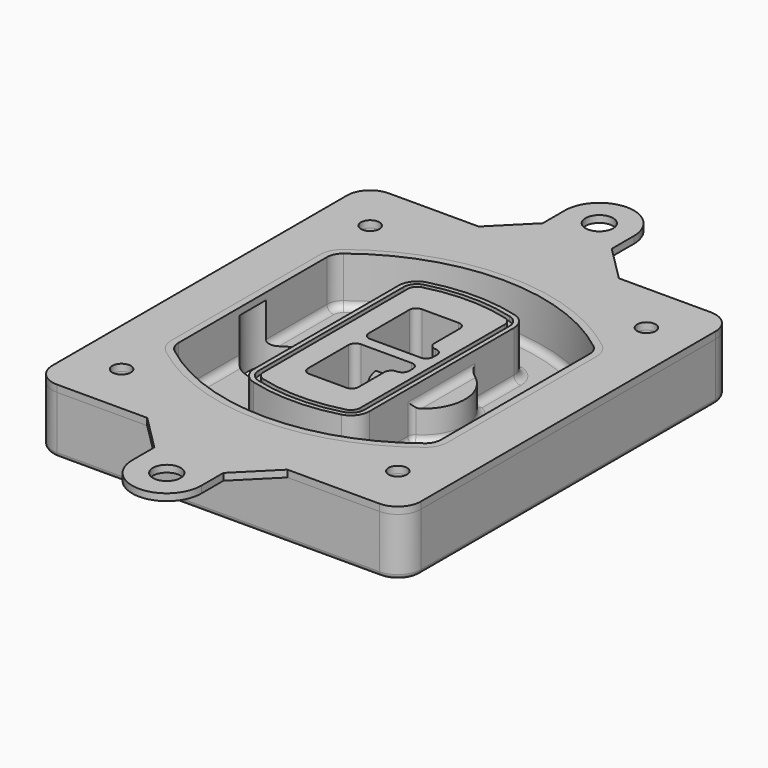
from build123d import *

# Parameters (mm, degrees)
F0_R      = 4
F1_DEPTH  = 25
F2_DEPTH  = 3
F3_DEPTH  = 18
F5_DEPTH  = 21
F6_DEPTH  = 2
F8_DEPTH  = 20
F9_DEPTH  = 16
F10_DEPTH = 25
F7_R      = 6
F7_R_2    = 4
F11_DEPTH = 6
F13_DEPTH = 9
F14_R     = 3
F15_R     = 2
F16_R     = 4
F16_R_2   = 6
F17_DEPTH = 3


# Not quite as in the source:
# - a feature names something its author has since deleted; it is built from what else it names


with BuildPart() as f1:
    # F0 (on Top) → F1 (new body)
    with BuildSketch(Plane.XY):
        with BuildLine():
            ThreePointArc((-80, -80), (-77.0710678119, -87.0710678119), (-70, -90))
            Line((-70, -90), (70, -90))
            ThreePointArc((70, -90), (77.0710678119, -87.0710678119), (80, -80))
            Line((80, -80), (80, 80))
            ThreePointArc((80, 80), (77.0710678119, 87.0710678119), (70, 90))
            Line((70, 90), (-70, 90))
            ThreePointArc((-70, 90), (-77.0710678119, 87.0710678119), (-80, 80))
            Line((-80, 80), (-80, -80))
        make_face()
        with Locations((-60, -67.5)):
            Circle(F0_R, mode=Mode.SUBTRACT)
        with Locations((60, -67.5)):
            Circle(F0_R, mode=Mode.SUBTRACT)
        with Locations((-60, 67.5)):
            Circle(F0_R, mode=Mode.SUBTRACT)
        with BuildLine():
            ThreePointArc((-64, 40.2934422872), (-62.5820384798, 46.4328484224), (-58.6153846154, 51.3286200352))
            ThreePointArc((-58.6153846154, 51.3286200352), (0, 71.5), (58.6153846154, 51.3286200352))
            ThreePointArc((58.6153846154, 51.3286200352), (62.5820384798, 46.4328484224), (64, 40.2934422872))
            Line((64, 40.2934422872), (64, -40.2934422872))
            ThreePointArc((64, -40.2934422872), (62.5820384798, -46.4328484224), (58.6153846154, -51.3286200352))
            ThreePointArc((58.6153846154, -51.3286200352), (0, -71.5), (-58.6153846154, -51.3286200352))
            ThreePointArc((-58.6153846154, -51.3286200352), (-62.5820384798, -46.4328484224), (-64, -40.2934422872))
            Line((-64, -40.2934422872), (-64, 40.2934422872))
        make_face(mode=Mode.SUBTRACT)
        with Locations((60, 67.5)):
            Circle(F0_R, mode=Mode.SUBTRACT)
        with BuildLine():
            ThreePointArc((58.6153846154, 51.3286200352), (0, 71.5), (-58.6153846154, 51.3286200352))
            ThreePointArc((-58.6153846154, 51.3286200352), (-62.5820384798, 46.4328484224), (-64, 40.2934422872))
            Line((-64, 40.2934422872), (-64, -40.2934422872))
            ThreePointArc((-64, -40.2934422872), (-62.5820384798, -46.4328484224), (-58.6153846154, -51.3286200352))
            ThreePointArc((-58.6153846154, -51.3286200352), (0, -71.5), (58.6153846154, -51.3286200352))
            ThreePointArc((58.6153846154, -51.3286200352), (62.5820384798, -46.4328484224), (64, -40.2934422872))
            Line((64, -40.2934422872), (64, 40.2934422872))
            ThreePointArc((64, 40.2934422872), (62.5820384798, 46.4328484224), (58.6153846154, 51.3286200352))
        make_face()
        with BuildLine():
            Line((-60, -40.2934422872), (-60, 40.2934422872))
            ThreePointArc((-60, 40.2934422872), (-58.9871703427, 44.6787323838), (-56.1538461538, 48.1757121072))
            ThreePointArc((-56.1538461538, 48.1757121072), (0, 67.5), (56.1538461538, 48.1757121072))
            ThreePointArc((56.1538461538, 48.1757121072), (58.9871703427, 44.6787323838), (60, 40.2934422872))
            Line((60, 40.2934422872), (60, -40.2934422872))
            ThreePointArc((60, -40.2934422872), (58.9871703427, -44.6787323838), (56.1538461538, -48.1757121072))
            ThreePointArc((56.1538461538, -48.1757121072), (0, -67.5), (-56.1538461538, -48.1757121072))
            ThreePointArc((-56.1538461538, -48.1757121072), (-58.9871703427, -44.6787323838), (-60, -40.2934422872))
        make_face(mode=Mode.SUBTRACT)
        with BuildLine():
            ThreePointArc((-56.1538461538, 48.1757121072), (-58.9871703427, 44.6787323838), (-60, 40.2934422872))
            Line((-60, 40.2934422872), (-60, -40.2934422872))
            ThreePointArc((-60, -40.2934422872), (-58.9871703427, -44.6787323838), (-56.1538461538, -48.1757121072))
            ThreePointArc((-56.1538461538, -48.1757121072), (0, -67.5), (56.1538461538, -48.1757121072))
            ThreePointArc((56.1538461538, -48.1757121072), (58.9871703427, -44.6787323838), (60, -40.2934422872))
            Line((60, -40.2934422872), (60, 40.2934422872))
            ThreePointArc((60, 40.2934422872), (58.9871703427, 44.6787323838), (56.1538461538, 48.1757121072))
            ThreePointArc((56.1538461538, 48.1757121072), (0, 67.5), (-56.1538461538, 48.1757121072))
        make_face()
        with BuildLine():
            ThreePointArc((54.3076923077, 45.8110311612), (56.2910192399, 43.3631453548), (57, 40.2934422872))
            Line((57, 40.2934422872), (57, -40.2934422872))
            ThreePointArc((57, -40.2934422872), (56.2910192399, -43.3631453548), (54.3076923077, -45.8110311612))
            ThreePointArc((54.3076923077, -45.8110311612), (0, -64.5), (-54.3076923077, -45.8110311612))
            ThreePointArc((-54.3076923077, -45.8110311612), (-56.2910192399, -43.3631453548), (-57, -40.2934422872))
            Line((-57, -40.2934422872), (-57, 40.2934422872))
            ThreePointArc((-57, 40.2934422872), (-56.2910192399, 43.3631453548), (-54.3076923077, 45.8110311612))
            ThreePointArc((-54.3076923077, 45.8110311612), (0, 64.5), (54.3076923077, 45.8110311612))
        make_face(mode=Mode.SUBTRACT)
        with BuildLine():
            Line((57, -40.2934422872), (57, 40.2934422872))
            ThreePointArc((57, 40.2934422872), (56.2910192399, 43.3631453548), (54.3076923077, 45.8110311612))
            ThreePointArc((54.3076923077, 45.8110311612), (0, 64.5), (-54.3076923077, 45.8110311612))
            ThreePointArc((-54.3076923077, 45.8110311612), (-56.2910192399, 43.3631453548), (-57, 40.2934422872))
            Line((-57, 40.2934422872), (-57, -40.2934422872))
            ThreePointArc((-57, -40.2934422872), (-56.2910192399, -43.3631453548), (-54.3076923077, -45.8110311612))
            ThreePointArc((-54.3076923077, -45.8110311612), (0, -64.5), (54.3076923077, -45.8110311612))
            ThreePointArc((54.3076923077, -45.8110311612), (56.2910192399, -43.3631453548), (57, -40.2934422872))
        make_face()
    extrude(amount=-F1_DEPTH)

    # F0 (on Top) → F2 (join)
    with BuildSketch(Plane.XY):
        with BuildLine():
            ThreePointArc((-56.1538461538, 48.1757121072), (-58.9871703427, 44.6787323838), (-60, 40.2934422872))
            Line((-60, 40.2934422872), (-60, -40.2934422872))
            ThreePointArc((-60, -40.2934422872), (-58.9871703427, -44.6787323838), (-56.1538461538, -48.1757121072))
            ThreePointArc((-56.1538461538, -48.1757121072), (0, -67.5), (56.1538461538, -48.1757121072))
            ThreePointArc((56.1538461538, -48.1757121072), (58.9871703427, -44.6787323838), (60, -40.2934422872))
            Line((60, -40.2934422872), (60, 40.2934422872))
            ThreePointArc((60, 40.2934422872), (58.9871703427, 44.6787323838), (56.1538461538, 48.1757121072))
            ThreePointArc((56.1538461538, 48.1757121072), (0, 67.5), (-56.1538461538, 48.1757121072))
        make_face()
        with BuildLine():
            ThreePointArc((54.3076923077, 45.8110311612), (56.2910192399, 43.3631453548), (57, 40.2934422872))
            Line((57, 40.2934422872), (57, -40.2934422872))
            ThreePointArc((57, -40.2934422872), (56.2910192399, -43.3631453548), (54.3076923077, -45.8110311612))
            ThreePointArc((54.3076923077, -45.8110311612), (0, -64.5), (-54.3076923077, -45.8110311612))
            ThreePointArc((-54.3076923077, -45.8110311612), (-56.2910192399, -43.3631453548), (-57, -40.2934422872))
            Line((-57, -40.2934422872), (-57, 40.2934422872))
            ThreePointArc((-57, 40.2934422872), (-56.2910192399, 43.3631453548), (-54.3076923077, 45.8110311612))
            ThreePointArc((-54.3076923077, 45.8110311612), (0, 64.5), (54.3076923077, 45.8110311612))
        make_face(mode=Mode.SUBTRACT)
    extrude(amount=F2_DEPTH)

    # F0 (on Top) → F3 (cut)
    with BuildSketch(Plane.XY):
        with BuildLine():
            Line((57, -40.2934422872), (57, 40.2934422872))
            ThreePointArc((57, 40.2934422872), (56.2910192399, 43.3631453548), (54.3076923077, 45.8110311612))
            ThreePointArc((54.3076923077, 45.8110311612), (0, 64.5), (-54.3076923077, 45.8110311612))
            ThreePointArc((-54.3076923077, 45.8110311612), (-56.2910192399, 43.3631453548), (-57, 40.2934422872))
            Line((-57, 40.2934422872), (-57, -40.2934422872))
            ThreePointArc((-57, -40.2934422872), (-56.2910192399, -43.3631453548), (-54.3076923077, -45.8110311612))
            ThreePointArc((-54.3076923077, -45.8110311612), (0, -64.5), (54.3076923077, -45.8110311612))
            ThreePointArc((54.3076923077, -45.8110311612), (56.2910192399, -43.3631453548), (57, -40.2934422872))
        make_face()
    extrude(amount=-F3_DEPTH, mode=Mode.SUBTRACT)

    # F4 (on face) → F5 (join, through all)
    with BuildSketch(Plane.XY.offset(3)):
        with BuildLine():
            ThreePointArc((-25, -39.2465276821), (-23.3511545998, -44.1109737193), (-19.0842911877, -46.9702398883))
            ThreePointArc((-19.0842911877, -46.9702398883), (0, -49.5), (19.0842911877, -46.9702398883))
            ThreePointArc((19.0842911877, -46.9702398883), (23.3511545998, -44.1109737193), (25, -39.2465276821))
            Line((25, -39.2465276821), (25, 39.2465276821))
            ThreePointArc((25, 39.2465276821), (23.3511545998, 44.1109737193), (19.0842911877, 46.9702398883))
            ThreePointArc((19.0842911877, 46.9702398883), (0, 49.5), (-19.0842911877, 46.9702398883))
            ThreePointArc((-19.0842911877, 46.9702398883), (-23.3511545998, 44.1109737193), (-25, 39.2465276821))
            Line((-25, 39.2465276821), (-25, -39.2465276821))
        make_face()
        with BuildLine():
            ThreePointArc((18.5632183908, 45.0393118368), (21.7633659499, 42.89486221), (23, 39.2465276821))
            Line((23, 39.2465276821), (23, -39.2465276821))
            ThreePointArc((23, -39.2465276821), (21.7633659499, -42.89486221), (18.5632183908, -45.0393118368))
            ThreePointArc((18.5632183908, -45.0393118368), (0, -47.5), (-18.5632183908, -45.0393118368))
            ThreePointArc((-18.5632183908, -45.0393118368), (-21.7633659499, -42.89486221), (-23, -39.2465276821))
            Line((-23, -39.2465276821), (-23, 39.2465276821))
            ThreePointArc((-23, 39.2465276821), (-21.7633659499, 42.89486221), (-18.5632183908, 45.0393118368))
            ThreePointArc((-18.5632183908, 45.0393118368), (0, 47.5), (18.5632183908, 45.0393118368))
        make_face(mode=Mode.SUBTRACT)
        with BuildLine():
            Line((23, -39.2465276821), (23, 39.2465276821))
            ThreePointArc((23, 39.2465276821), (21.7633659499, 42.89486221), (18.5632183908, 45.0393118368))
            ThreePointArc((18.5632183908, 45.0393118368), (0, 47.5), (-18.5632183908, 45.0393118368))
            ThreePointArc((-18.5632183908, 45.0393118368), (-21.7633659499, 42.89486221), (-23, 39.2465276821))
            Line((-23, 39.2465276821), (-23, -39.2465276821))
            ThreePointArc((-23, -39.2465276821), (-21.7633659499, -42.89486221), (-18.5632183908, -45.0393118368))
            ThreePointArc((-18.5632183908, -45.0393118368), (0, -47.5), (18.5632183908, -45.0393118368))
            ThreePointArc((18.5632183908, -45.0393118368), (21.7633659499, -42.89486221), (23, -39.2465276821))
        make_face()
        with BuildLine():
            ThreePointArc((18.0421455939, 43.1083837852), (20.1755772999, 41.6787507007), (21, 39.2465276821))
            Line((21, 39.2465276821), (21, -39.2465276821))
            ThreePointArc((21, -39.2465276821), (20.1755772999, -41.6787507007), (18.0421455939, -43.1083837852))
            ThreePointArc((18.0421455939, -43.1083837852), (0, -45.5), (-18.0421455939, -43.1083837852))
            ThreePointArc((-18.0421455939, -43.1083837852), (-20.1755772999, -41.6787507007), (-21, -39.2465276821))
            Line((-21, -39.2465276821), (-21, 39.2465276821))
            ThreePointArc((-21, 39.2465276821), (-20.1755772999, 41.6787507007), (-18.0421455939, 43.1083837852))
            ThreePointArc((-18.0421455939, 43.1083837852), (0, 45.5), (18.0421455939, 43.1083837852))
        make_face(mode=Mode.SUBTRACT)
        with BuildLine():
            Line((21, -39.2465276821), (21, 39.2465276821))
            ThreePointArc((21, 39.2465276821), (20.1755772999, 41.6787507007), (18.0421455939, 43.1083837852))
            ThreePointArc((18.0421455939, 43.1083837852), (0, 45.5), (-18.0421455939, 43.1083837852))
            ThreePointArc((-18.0421455939, 43.1083837852), (-20.1755772999, 41.6787507007), (-21, 39.2465276821))
            Line((-21, 39.2465276821), (-21, -39.2465276821))
            ThreePointArc((-21, -39.2465276821), (-20.1755772999, -41.6787507007), (-18.0421455939, -43.1083837852))
            ThreePointArc((-18.0421455939, -43.1083837852), (0, -45.5), (18.0421455939, -43.1083837852))
            ThreePointArc((18.0421455939, -43.1083837852), (20.1755772999, -41.6787507007), (21, -39.2465276821))
        make_face()
        with BuildLine():
            Line((-8, -2.5), (14, -2.5))
            ThreePointArc((14, -2.5), (16.1213203436, -3.3786796564), (17, -5.5))
            Line((17, -5.5), (17, -7.5))
            ThreePointArc((17, -7.5), (16.1213203436, -9.6213203436), (14, -10.5))
            ThreePointArc((14, -10.5), (11.8786796564, -11.3786796564), (11, -13.5))
            Line((11, -13.5), (11, -27.5))
            ThreePointArc((11, -27.5), (10.1213203436, -29.6213203436), (8, -30.5))
            Line((8, -30.5), (-8, -30.5))
            ThreePointArc((-8, -30.5), (-10.1213203436, -29.6213203436), (-11, -27.5))
            Line((-11, -27.5), (-11, -5.5))
            ThreePointArc((-11, -5.5), (-10.1213203436, -3.3786796564), (-8, -2.5))
        make_face(mode=Mode.SUBTRACT)
        with BuildLine():
            ThreePointArc((-8, 2.5), (-10.1213203436, 3.3786796564), (-11, 5.5))
            Line((-11, 5.5), (-11, 27.5))
            ThreePointArc((-11, 27.5), (-10.1213203436, 29.6213203436), (-8, 30.5))
            Line((-8, 30.5), (8, 30.5))
            ThreePointArc((8, 30.5), (10.1213203436, 29.6213203436), (11, 27.5))
            Line((11, 27.5), (11, 13.5))
            ThreePointArc((11, 13.5), (11.8786796564, 11.3786796564), (14, 10.5))
            ThreePointArc((14, 10.5), (16.1213203436, 9.6213203436), (17, 7.5))
            Line((17, 7.5), (17, 5.5))
            ThreePointArc((17, 5.5), (16.1213203436, 3.3786796564), (14, 2.5))
            Line((14, 2.5), (-8, 2.5))
        make_face(mode=Mode.SUBTRACT)
    extrude(amount=-F5_DEPTH)

    # F4 (on face) → F6 (cut)
    with BuildSketch(Plane.XY.offset(3)):
        with BuildLine():
            Line((23, -39.2465276821), (23, 39.2465276821))
            ThreePointArc((23, 39.2465276821), (21.7633659499, 42.89486221), (18.5632183908, 45.0393118368))
            ThreePointArc((18.5632183908, 45.0393118368), (0, 47.5), (-18.5632183908, 45.0393118368))
            ThreePointArc((-18.5632183908, 45.0393118368), (-21.7633659499, 42.89486221), (-23, 39.2465276821))
            Line((-23, 39.2465276821), (-23, -39.2465276821))
            ThreePointArc((-23, -39.2465276821), (-21.7633659499, -42.89486221), (-18.5632183908, -45.0393118368))
            ThreePointArc((-18.5632183908, -45.0393118368), (0, -47.5), (18.5632183908, -45.0393118368))
            ThreePointArc((18.5632183908, -45.0393118368), (21.7633659499, -42.89486221), (23, -39.2465276821))
        make_face()
        with BuildLine():
            ThreePointArc((18.0421455939, 43.1083837852), (20.1755772999, 41.6787507007), (21, 39.2465276821))
            Line((21, 39.2465276821), (21, -39.2465276821))
            ThreePointArc((21, -39.2465276821), (20.1755772999, -41.6787507007), (18.0421455939, -43.1083837852))
            ThreePointArc((18.0421455939, -43.1083837852), (0, -45.5), (-18.0421455939, -43.1083837852))
            ThreePointArc((-18.0421455939, -43.1083837852), (-20.1755772999, -41.6787507007), (-21, -39.2465276821))
            Line((-21, -39.2465276821), (-21, 39.2465276821))
            ThreePointArc((-21, 39.2465276821), (-20.1755772999, 41.6787507007), (-18.0421455939, 43.1083837852))
            ThreePointArc((-18.0421455939, 43.1083837852), (0, 45.5), (18.0421455939, 43.1083837852))
        make_face(mode=Mode.SUBTRACT)
    extrude(amount=-F6_DEPTH, mode=Mode.SUBTRACT)

    # F7 (on face) → F8 (join)
    with BuildSketch(Plane(origin=(0, 0, -25), x_dir=(1, 0, 0), z_dir=(0, 0, -1))):
        with BuildLine():
            ThreePointArc((3.28842436, 0), (16.7567035675, 13.4682792075), (30.224982775, 0))
            Line((30.224982775, 0), (35.224982775, 0))
            ThreePointArc((35.224982775, 0), (16.7567035675, 18.4682792075), (-1.71157564, 0))
            Line((-1.71157564, 0), (3.28842436, 0))
        make_face()
        with BuildLine():
            Line((3.28842436, 0), (30.224982775, 0))
            ThreePointArc((30.224982775, 0), (16.7567035675, 13.4682792075), (3.28842436, 0))
        make_face()
        with BuildLine():
            ThreePointArc((3.28842436, 0), (16.7567035675, -13.4682792075), (30.224982775, 0))
            Line((30.224982775, 0), (3.28842436, 0))
        make_face()
        with BuildLine():
            Line((35.224982775, 0), (30.224982775, 0))
            ThreePointArc((30.224982775, 0), (16.7567035675, -13.4682792075), (3.28842436, 0))
            Line((3.28842436, 0), (-1.71157564, 0))
            ThreePointArc((-1.71157564, 0), (16.7567035675, -18.4682792075), (35.224982775, 0))
        make_face()
    extrude(amount=-F8_DEPTH)

    # F7 (on face) → F9 (cut)
    with BuildSketch(Plane(origin=(0, 0, -25), x_dir=(1, 0, 0), z_dir=(0, 0, -1))):
        with BuildLine():
            Line((3.28842436, 0), (30.224982775, 0))
            ThreePointArc((30.224982775, 0), (16.7567035675, 13.4682792075), (3.28842436, 0))
        make_face()
        with BuildLine():
            ThreePointArc((3.28842436, 0), (16.7567035675, -13.4682792075), (30.224982775, 0))
            Line((30.224982775, 0), (3.28842436, 0))
        make_face()
    extrude(amount=-F9_DEPTH, mode=Mode.SUBTRACT)

    # F7 (on face) → F10 (cut)
    with BuildSketch(Plane(origin=(0, 0, -25), x_dir=(1, 0, 0), z_dir=(0, 0, -1))):
        with BuildLine():
            Line((-59.0318229325, 0), (-32.0952645175, 0))
            ThreePointArc((-32.0952645175, 0), (-45.563543725, 13.4682792075), (-59.0318229325, 0))
        make_face()
        with BuildLine():
            ThreePointArc((-59.0318229325, 0), (-45.563543725, -13.4682792075), (-32.0952645175, 0))
            Line((-32.0952645175, 0), (-59.0318229325, 0))
        make_face()
    extrude(amount=-F10_DEPTH, mode=Mode.SUBTRACT)

    # F7 (on face) → F11 (cut)
    with BuildSketch(Plane(origin=(0, 0, -25), x_dir=(1, 0, 0), z_dir=(0, 0, -1))):
        with Locations((60, -67.5)):
            Circle(F7_R)
        with Locations((60, -67.5)):
            Circle(F7_R_2, mode=Mode.SUBTRACT)
        with Locations((-60, -67.5)):
            Circle(F7_R)
        with Locations((-60, -67.5)):
            Circle(F7_R_2, mode=Mode.SUBTRACT)
        with Locations((-60, 67.5)):
            Circle(F7_R)
        with Locations((-60, 67.5)):
            Circle(F7_R_2, mode=Mode.SUBTRACT)
        with Locations((60, 67.5)):
            Circle(F7_R)
        with Locations((60, 67.5)):
            Circle(F7_R_2, mode=Mode.SUBTRACT)
    extrude(amount=-F11_DEPTH, mode=Mode.SUBTRACT)

    # F12 (on face) → F13 (cut, through all)
    with BuildSketch(Plane(origin=(0, 0, -9), x_dir=(1, 0, 0), z_dir=(0, 0, -1))):
        with BuildLine():
            Line((11, 13.5), (11, 17.5481537753))
            ThreePointArc((11, 17.5481537753), (2.5696536419, 11.8239143813), (-1.5415842455, 2.5))
            Line((-1.5415842455, 2.5), (3.5224848595, 2.5))
            ThreePointArc((3.5224848595, 2.5), (6.1857188154, 8.3455872281), (11.2536447004, 12.2927168648))
            ThreePointArc((11.2536447004, 12.2927168648), (11.0640958889, 12.8831798879), (11, 13.5))
        make_face()
        with BuildLine():
            ThreePointArc((11.2536447004, -12.2927168648), (6.1857188154, -8.3455872281), (3.5224848595, -2.5))
            Line((3.5224848595, -2.5), (-1.5415842455, -2.5))
            ThreePointArc((-1.5415842455, -2.5), (2.5696536419, -11.8239143813), (11, -17.5481537753))
            Line((11, -17.5481537753), (11, -13.5))
            ThreePointArc((11, -13.5), (11.0640958889, -12.8831798879), (11.2536447004, -12.2927168648))
        make_face()
        with BuildLine():
            ThreePointArc((11.2536447004, 12.2927168648), (6.1857188154, 8.3455872281), (3.5224848595, 2.5))
            Line((3.5224848595, 2.5), (14, 2.5))
            ThreePointArc((14, 2.5), (16.1213203436, 3.3786796564), (17, 5.5))
            Line((17, 5.5), (17, 7.5))
            ThreePointArc((17, 7.5), (16.1213203436, 9.6213203436), (14, 10.5))
            ThreePointArc((14, 10.5), (12.3601599782, 10.9878446101), (11.2536447004, 12.2927168648))
        make_face()
        with BuildLine():
            Line((14, -2.5), (3.5224848595, -2.5))
            ThreePointArc((3.5224848595, -2.5), (6.1857188154, -8.3455872281), (11.2536447004, -12.2927168648))
            ThreePointArc((11.2536447004, -12.2927168648), (12.3601599782, -10.9878446101), (14, -10.5))
            ThreePointArc((14, -10.5), (16.1213203436, -9.6213203436), (17, -7.5))
            Line((17, -7.5), (17, -5.5))
            ThreePointArc((17, -5.5), (16.1213203436, -3.3786796564), (14, -2.5))
        make_face()
    extrude(amount=F13_DEPTH, mode=Mode.SUBTRACT)

    # F14
    f14_edges = [f1.edges().sort_by_distance(p)[0] for p in [
        (-57, -23.703476, -18),
        (-57, 23.703476, -18),
        (25, 0, -5),
        (25, 16.526506, -11.5),
        (25, -16.526506, -11.5),
        (25, -27.886517, -18),
        (35.224983, 0, -18),
    ]]
    fillet(f14_edges, radius=F14_R)

    # F15
    f15_edges = [f1.edges().sort_by_distance(p)[0] for p in [
        (0, -90, -25),
    ]]
    fillet(f15_edges, radius=F15_R)


with BuildPart() as f17:
    # F16 (on face) → F17 (new body, through all)
    with BuildSketch(Plane.XY):
        with BuildLine():
            Line((30.025821902, 90), (-30.8484099805, 90))
            Line((-30.8484099805, 90), (-70, 90))
            ThreePointArc((-70, 90), (-77.0710678119, 87.0710678119), (-80, 80))
            Line((-80, 80), (-80, 0))
            Line((-80, 0), (-60, 0))
            Line((-60, 0), (-60, 40.2934422872))
            ThreePointArc((-60, 40.2934422872), (-58.9871703427, 44.6787323838), (-56.1538461538, 48.1757121072))
            ThreePointArc((-56.1538461538, 48.1757121072), (0, 67.5), (56.1538461538, 48.1757121072))
            ThreePointArc((56.1538461538, 48.1757121072), (58.9871703427, 44.6787323838), (60, 40.2934422872))
            Line((60, 40.2934422872), (60, 0))
            Line((60, 0), (80, 0))
            Line((80, 0), (80, 80))
            ThreePointArc((80, 80), (77.0710678119, 87.0710678119), (70, 90))
            Line((70, 90), (30.025821902, 90))
        make_face()
        with Locations((-60, 67.5)):
            Circle(F16_R, mode=Mode.SUBTRACT)
        with Locations((60, 67.5)):
            Circle(F16_R, mode=Mode.SUBTRACT)
        with BuildLine():
            Line((-60, 0), (-80, 0))
            Line((-80, 0), (-80, -80))
            ThreePointArc((-80, -80), (-77.0710678119, -87.0710678119), (-70, -90))
            Line((-70, -90), (-30.8484099805, -90))
            Line((-30.8484099805, -90), (30.025821902, -90))
            Line((30.025821902, -90), (70, -90))
            ThreePointArc((70, -90), (77.0710678119, -87.0710678119), (80, -80))
            Line((80, -80), (80, 0))
            Line((80, 0), (60, 0))
            Line((60, 0), (60, -40.2934422872))
            ThreePointArc((60, -40.2934422872), (58.9871703427, -44.6787323838), (56.1538461538, -48.1757121072))
            ThreePointArc((56.1538461538, -48.1757121072), (0, -67.5), (-56.1538461538, -48.1757121072))
            ThreePointArc((-56.1538461538, -48.1757121072), (-58.9871703427, -44.6787323838), (-60, -40.2934422872))
            Line((-60, -40.2934422872), (-60, 0))
        make_face()
        with Locations((-60, -67.5)):
            Circle(F16_R, mode=Mode.SUBTRACT)
        with Locations((60, -67.5)):
            Circle(F16_R, mode=Mode.SUBTRACT)
        with BuildLine():
            Line((-15.4112940393, 117.4371159413), (-15.4112940393, 105.4371159413))
            Line((-15.4112940393, 105.4371159413), (-30.8484099805, 90))
            Line((-30.8484099805, 90), (30.025821902, 90))
            Line((30.025821902, 90), (14.5887059607, 105.4371159413))
            Line((14.5887059607, 105.4371159413), (14.5887059607, 117.4371159413))
            ThreePointArc((14.5887059607, 117.4371159413), (-0.4112940393, 132.4371159413), (-15.4112940393, 117.4371159413))
        make_face()
        with Locations((-0.4112940393, 117.4371159413)):
            Circle(F16_R_2, mode=Mode.SUBTRACT)
        with BuildLine():
            Line((30.025821902, -90), (-30.8484099805, -90))
            Line((-30.8484099805, -90), (-15.4112940393, -105.4371159413))
            Line((-15.4112940393, -105.4371159413), (-15.4112940393, -117.4371159413))
            ThreePointArc((-15.4112940393, -117.4371159413), (-0.4112940393, -132.4371159413), (14.5887059607, -117.4371159413))
            Line((14.5887059607, -117.4371159413), (14.5887059607, -105.4371159413))
            Line((14.5887059607, -105.4371159413), (30.025821902, -90))
        make_face()
        with Locations((-0.4112940393, -117.4371159413)):
            Circle(F16_R_2, mode=Mode.SUBTRACT)
    extrude(amount=F17_DEPTH)


solid = Compound([f1.part, f17.part])
